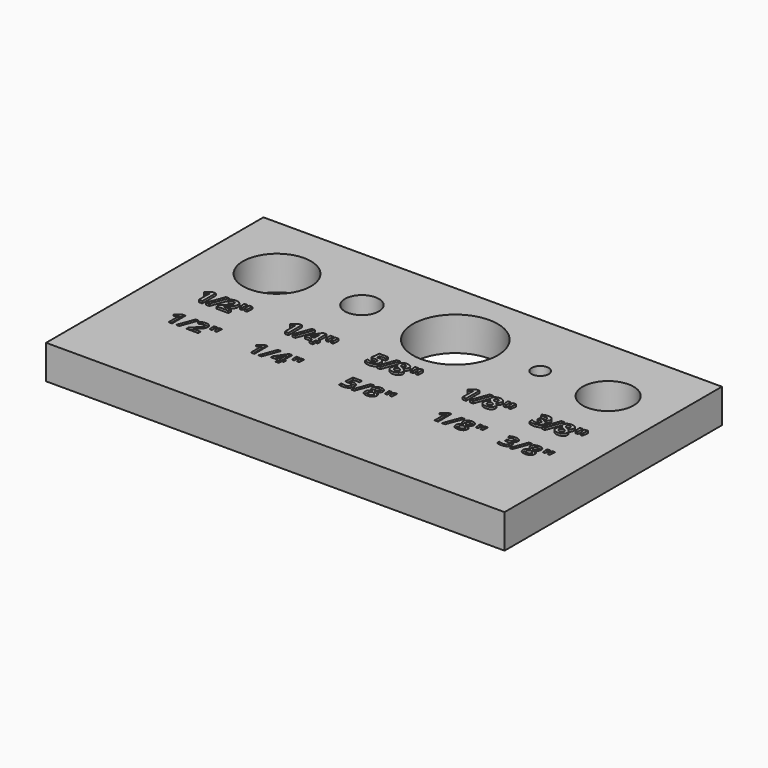
from build123d import *

# Parameters (mm, degrees)
F0_W         = 85.725
F0_H         = 50.8
F0_R         = 6.35
F0_R_2       = 3.175
F0_R_3       = 7.9375
F0_R_4       = 1.5875
F0_R_5       = 4.7625
F1_DEPTH     = 6.35
F2_TEXT_SIZE = 4.4097222222
F4_DEPTH     = 0.396875
F3_TEXT_SIZE = 4.4097222222
F5_DEPTH     = 0.396875


# Not quite as in the source:
# - Text() gives the source's letters only with a copy of the font that has no kerning and outlines rounded to 1/6400 em; it was checked with that copy


with BuildPart() as f1:
    # F0 (on Top) → F1 (new body)
    with BuildSketch(Plane.XY):
        with Locations((-42.8625, 25.4)):
            Rectangle(F0_W, F0_H)
        with Locations((-73.025, 38.1)):
            Circle(F0_R, mode=Mode.SUBTRACT)
        with Locations((-57.15, 38.1)):
            Circle(F0_R_2, mode=Mode.SUBTRACT)
        with Locations((-39.6875, 38.1)):
            Circle(F0_R_3, mode=Mode.SUBTRACT)
        with Locations((-23.8125, 38.1)):
            Circle(F0_R_4, mode=Mode.SUBTRACT)
        with Locations((-11.1125, 38.1)):
            Circle(F0_R_5, mode=Mode.SUBTRACT)
    extrude(amount=F1_DEPTH)

    # F2 (on face) → F4 (join)
    with BuildSketch(Plane.XY.offset(6.35)):
        with Locations((-77.493633355, 23.9476066638)):
            Text('1/2"', F2_TEXT_SIZE, font='Open Sans', font_style=FontStyle.BOLD, text_align=(TextAlign.LEFT, TextAlign.BOTTOM))
        with Locations((-14.7410290573, 23.9476066638)):
            Text('3/8"', F2_TEXT_SIZE, font='Open Sans', font_style=FontStyle.BOLD, text_align=(TextAlign.LEFT, TextAlign.BOTTOM))
        with Locations((-45.5386079086, 23.9476066638)):
            Text('5/8"', F2_TEXT_SIZE, font='Open Sans', font_style=FontStyle.BOLD, text_align=(TextAlign.LEFT, TextAlign.BOTTOM))
        with Locations((-61.4011400235, 23.9476066638)):
            Text('1/4"', F2_TEXT_SIZE, font='Open Sans', font_style=FontStyle.BOLD, text_align=(TextAlign.LEFT, TextAlign.BOTTOM))
        with Locations((-28.1825753619, 23.9476066638)):
            Text('1/8"', F2_TEXT_SIZE, font='Open Sans', font_style=FontStyle.BOLD, text_align=(TextAlign.LEFT, TextAlign.BOTTOM))
    extrude(amount=F4_DEPTH)

    # F3 (on face) → F5 (cut)
    with BuildSketch(Plane.XY.offset(6.35)):
        with Locations((-76.996381606, 16.2574294955)):
            Text('1/2"', F3_TEXT_SIZE, font='Open Sans', font_style=FontStyle.BOLD, text_align=(TextAlign.LEFT, TextAlign.BOTTOM))
        with Locations((-14.6986026574, 16.2574294955)):
            Text('3/8"', F3_TEXT_SIZE, font='Open Sans', font_style=FontStyle.BOLD, text_align=(TextAlign.LEFT, TextAlign.BOTTOM))
        with Locations((-44.2524104548, 16.2574294955)):
            Text('5/8"', F3_TEXT_SIZE, font='Open Sans', font_style=FontStyle.BOLD, text_align=(TextAlign.LEFT, TextAlign.BOTTOM))
        with Locations((-61.6074764025, 16.2574294955)):
            Text('1/4"', F3_TEXT_SIZE, font='Open Sans', font_style=FontStyle.BOLD, text_align=(TextAlign.LEFT, TextAlign.BOTTOM))
        with Locations((-27.269516023, 16.2574294955)):
            Text('1/8"', F3_TEXT_SIZE, font='Open Sans', font_style=FontStyle.BOLD, text_align=(TextAlign.LEFT, TextAlign.BOTTOM))
    extrude(amount=-F5_DEPTH, mode=Mode.SUBTRACT)


solid = f1.part
